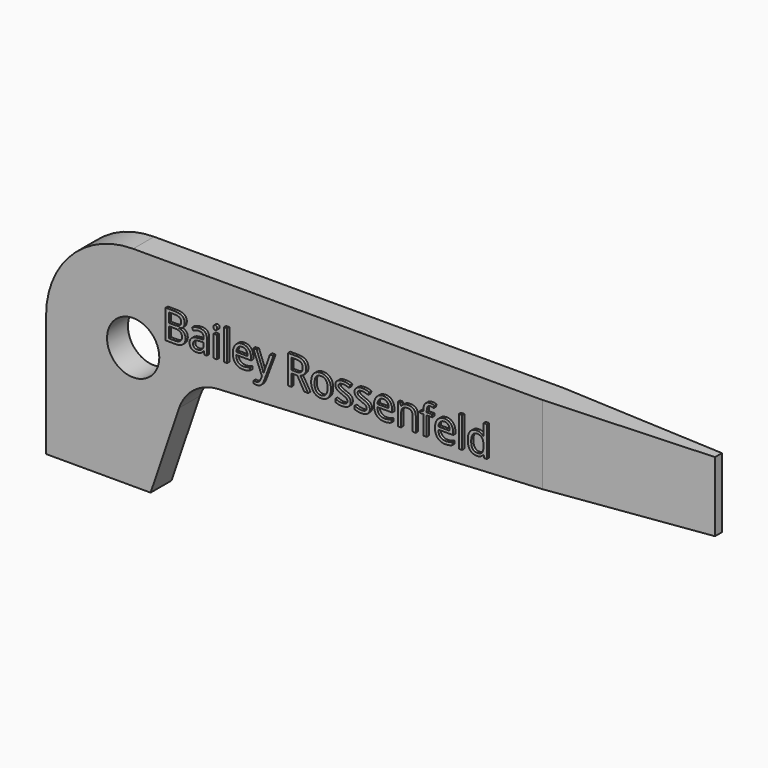
from build123d import *

# Parameters (mm, degrees)
F1_DEPTH     = 2.38125
F2_R         = 2.38125
F3_DEPTH     = 2.38225
F5_DEPTH     = 25.4
F6_TEXT_SIZE = 3.6733486141
F7_DEPTH     = 0.254


# Not quite as in the source:
# - Text() gives the source's letters only with a copy of the font that has no kerning and outlines rounded to 1/6400 em; it was checked with that copy


with BuildPart() as f1:
    # F0 (on Front) → F1 (new body)
    with BuildSketch(Plane.XZ):
        with BuildLine():
            Line((60.325, 19.05), (7.9375, 19.05))
            ThreePointArc((7.9375, 19.05), (2.3248399243, 16.7251600757), (0, 11.1125))
            Line((0, 11.1125), (0, 0))
            Line((0, 0), (9.525, 0))
            Line((9.525, 0), (12.1173647876, 7.6271664624))
            ThreePointArc((12.1173647876, 7.6271664624), (13.4786145605, 9.5135918491), (15.6631963617, 10.3130942181))
            Line((15.6631963617, 10.3130942181), (60.325, 12.7))
            Line((60.325, 12.7), (60.325, 19.05))
        make_face()
    extrude(amount=F1_DEPTH)

    # F2 (on face) → F3 (cut, through all)
    with BuildSketch(Plane.XZ.offset(2.38125)):
        with Locations((7.9375, 11.1125)):
            Circle(F2_R)
    extrude(amount=-F3_DEPTH, mode=Mode.SUBTRACT)

    # F4 (on face) → F5 (cut)
    with BuildSketch(Plane.XY.offset(19.05)):
        Polygon((60.325, 0), (45.24375, 0), (60.325, -0.79375), align=None)
        Polygon((60.325, -2.38125), (60.325, -1.5875), (45.24375, -2.38125), align=None)
    extrude(amount=-F5_DEPTH, mode=Mode.SUBTRACT)

    # F6 (on face) → F7 (join)
    with BuildSketch(Plane.XZ.offset(2.38125)):
        with Locations((10.7368901372, 12.8271877766)):
            Text('Bailey Rossenfeld', F6_TEXT_SIZE, font='Open Sans', text_align=(TextAlign.LEFT, TextAlign.BOTTOM))
    extrude(amount=F7_DEPTH)


solid = f1.part
